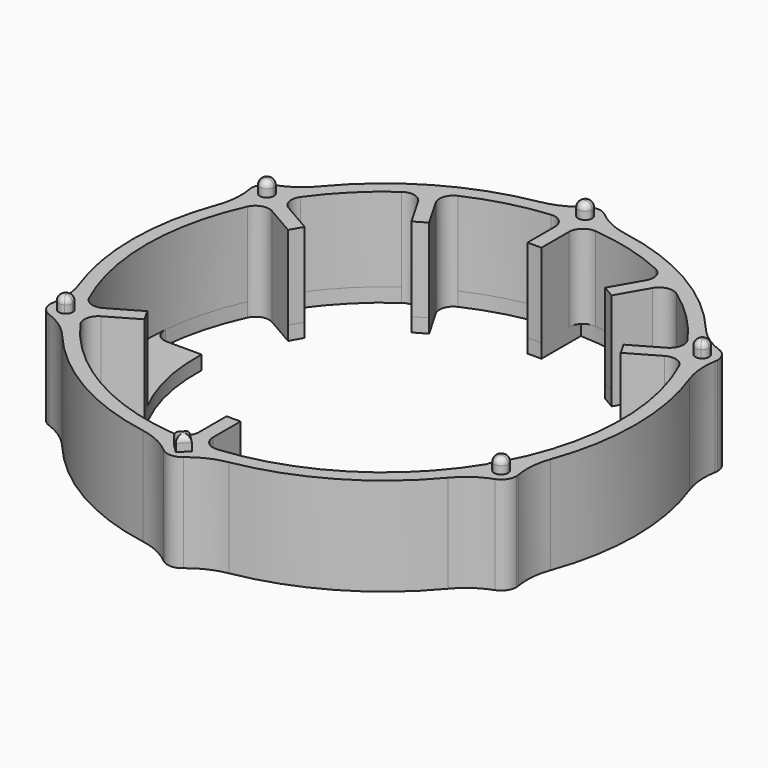
from build123d import *

# Parameters (mm, degrees)
F1_R         = 18
F1_R_2       = 17
F2_DEPTH     = 7
F3_DEPTH     = 7
F4_DEPTH     = 1
F6_DEPTH     = 7
F7_R         = 1
F8_R         = 5
F9_DEPTH     = 8
F10_R        = 0.44999
F11_DEPTH    = 1.8
F12_R        = 13.47
F13_DEPTH    = 1
F14_DEPTH    = 1
F15_T1_DEPTH = 3.7395798703
F15_T3_DEPTH = 1


# Not quite as in the source:
# - a fillet or chamfer that OpenCascade refuses, or shapes differently, is made with other operations: its cross-section is extruded or revolved along the edge and cut away or added
# - a fillet or chamfer is up to 0.001 mm smaller than in the source, because OpenCascade refuses the exact size
# - after a boolean that leaves OpenCascade's solid faulty, fix() repairs it


with BuildPart() as f2:
    # F1 (on Top) → F2 (new body)
    with BuildSketch(Plane.XY):
        Circle(F1_R)
        Circle(F1_R_2, mode=Mode.SUBTRACT)
    extrude(amount=F2_DEPTH)

    # F0 (on Top) → F3 (join)
    with BuildSketch(Plane.XY):
        with BuildLine():
            Line((-11.4073228059, 7.1633711619), (-14.4660626528, 8.9293354359))
            ThreePointArc((-14.4660626528, 8.9293354359), (-14.7224318643, 8.5), (-14.9660626528, 8.0633100321))
            Line((-14.9660626528, 8.0633100321), (-11.9073228059, 6.2973457581))
            ThreePointArc((-11.9073228059, 6.2973457581), (-11.665362189, 6.735), (-11.4073228059, 7.1633711619))
        make_face()
        with BuildLine():
            Line((7.1633711619, 11.4073228059), (8.9293354359, 14.4660626528))
            ThreePointArc((8.9293354359, 14.4660626528), (8.5, 14.7224318643), (8.0633100321, 14.9660626528))
            Line((8.0633100321, 14.9660626528), (6.2973457581, 11.9073228059))
            ThreePointArc((6.2973457581, 11.9073228059), (6.735, 11.665362189), (7.1633711619, 11.4073228059))
        make_face()
        with BuildLine():
            ThreePointArc((-0.5, -16.992645468), (0, -17), (0.5, -16.992645468))
            Line((0.5, -16.992645468), (0.5, -13.46071692))
            ThreePointArc((0.5, -13.46071692), (0, -13.47), (-0.5, -13.46071692))
            Line((-0.5, -13.46071692), (-0.5, -16.992645468))
        make_face()
        with BuildLine():
            ThreePointArc((-14.9660626528, -8.0633100321), (-14.7224318643, -8.5), (-14.4660626528, -8.9293354359))
            Line((-14.4660626528, -8.9293354359), (-11.4073228059, -7.1633711619))
            ThreePointArc((-11.4073228059, -7.1633711619), (-11.665362189, -6.735), (-11.9073228059, -6.2973457581))
            Line((-11.9073228059, -6.2973457581), (-14.9660626528, -8.0633100321))
        make_face()
        with BuildLine():
            Line((-6.2973457581, 11.9073228059), (-8.0633100321, 14.9660626528))
            ThreePointArc((-8.0633100321, 14.9660626528), (-8.5, 14.7224318643), (-8.9293354359, 14.4660626528))
            Line((-8.9293354359, 14.4660626528), (-7.1633711619, 11.4073228059))
            ThreePointArc((-7.1633711619, 11.4073228059), (-6.735, 11.665362189), (-6.2973457581, 11.9073228059))
        make_face()
        with BuildLine():
            Line((0.5, 13.46071692), (0.5, 16.992645468))
            ThreePointArc((0.5, 16.992645468), (0, 17), (-0.5, 16.992645468))
            Line((-0.5, 16.992645468), (-0.5, 13.46071692))
            ThreePointArc((-0.5, 13.46071692), (0, 13.47), (0.5, 13.46071692))
        make_face()
        with BuildLine():
            Line((11.9073228059, 6.2973457581), (14.9660626528, 8.0633100321))
            ThreePointArc((14.9660626528, 8.0633100321), (14.7224318643, 8.5), (14.4660626528, 8.9293354359))
            Line((14.4660626528, 8.9293354359), (11.4073228059, 7.1633711619))
            ThreePointArc((11.4073228059, 7.1633711619), (11.665362189, 6.735), (11.9073228059, 6.2973457581))
        make_face()
    extrude(amount=F3_DEPTH)

    # F1 (on Top) → F4 (join)
    with BuildSketch(Plane.XY):
        Circle(F1_R)
        Circle(F1_R_2, mode=Mode.SUBTRACT)
        Circle(F1_R_2)
    extrude(amount=F4_DEPTH)

    # F5 (on Top) → F6 (join)
    with BuildSketch(Plane.XY):
        with BuildLine():
            ThreePointArc((-14.4884572681, 9), (-14.6275367743, 9.5353800561), (-15.0096060035, 9.935377578))
            ThreePointArc((-15.0096060035, 9.935377578), (-15.1731450826, 9.6837837802), (-15.3324673166, 9.4294987133))
            ThreePointArc((-15.3324673166, 9.4294987133), (-15.153718855, 9.2469868663), (-15.0884572681, 9))
            ThreePointArc((-15.0884572681, 9), (-15.3354561915, 8.5687338928), (-15.832419089, 8.5635568422))
            ThreePointArc((-15.832419089, 8.5635568422), (-15.9729752997, 8.2984372068), (-16.1090923805, 8.0310113108))
            ThreePointArc((-16.1090923805, 8.0310113108), (-15.0239657375, 8.0558870238), (-14.4884572681, 9))
        make_face()
        with BuildLine():
            ThreePointArc((-15.3324673166, 9.4294987133), (-15.1731450826, 9.6837837802), (-15.0096060035, 9.935377578))
            ThreePointArc((-15.0096060035, 9.935377578), (-16.5410852123, 9.55), (-16.1090923805, 8.0310113108))
            ThreePointArc((-16.1090923805, 8.0310113108), (-15.9729752997, 8.2984372068), (-15.832419089, 8.5635568422))
            ThreePointArc((-15.832419089, 8.5635568422), (-16.02146997, 9.25), (-15.3324673166, 9.4294987133))
        make_face()
        with BuildLine():
            ThreePointArc((-1.099486377, 17.9663888889), (0, 16.9), (1.099486377, 17.9663888889))
            ThreePointArc((1.099486377, 17.9663888889), (0.7998302171, 17.982220987), (0.4999517724, 17.9930555556))
            ThreePointArc((0.4999517724, 17.9930555556), (0, 17.5), (-0.4999517724, 17.9930555556))
            ThreePointArc((-0.4999517724, 17.9930555556), (-0.7998302171, 17.982220987), (-1.099486377, 17.9663888889))
        make_face()
        with BuildLine():
            ThreePointArc((0.4999517724, 17.9930555556), (0.7998302171, 17.982220987), (1.099486377, 17.9663888889))
            ThreePointArc((1.099486377, 17.9663888889), (1.0998715868, 17.9831924823), (1.1, 18))
            ThreePointArc((1.1, 18), (-0.0168075177, 19.0998715868), (-1.099486377, 17.9663888889))
            ThreePointArc((-1.099486377, 17.9663888889), (-0.7998302171, 17.982220987), (-0.4999517724, 17.9930555556))
            ThreePointArc((-0.4999517724, 17.9930555556), (-0.003472306, 18.4999879429), (0.5, 18))
            ThreePointArc((0.5, 18), (0.4999879429, 17.996527694), (0.4999517724, 17.9930555556))
        make_face()
        with BuildLine():
            ThreePointArc((15.832419089, 8.5635568422), (15.9729752997, 8.2984372068), (16.1090923805, 8.0310113108))
            ThreePointArc((16.1090923805, 8.0310113108), (16.5325702443, 8.4355084694), (16.6884572681, 9))
            ThreePointArc((16.6884572681, 9), (16.1238373242, 9.9609204939), (15.0096060035, 9.935377578))
            ThreePointArc((15.0096060035, 9.935377578), (15.1731450826, 9.6837837802), (15.3324673166, 9.4294987133))
            ThreePointArc((15.3324673166, 9.4294987133), (15.8354441344, 9.4347384132), (16.0884572681, 9))
            ThreePointArc((16.0884572681, 9), (16.0197233753, 8.7469989234), (15.832419089, 8.5635568422))
        make_face()
        with BuildLine():
            ThreePointArc((15.0096060035, 9.935377578), (14.635829324, 8.45), (16.1090923805, 8.0310113108))
            ThreePointArc((16.1090923805, 8.0310113108), (15.9729752997, 8.2984372068), (15.832419089, 8.5635568422))
            ThreePointArc((15.832419089, 8.5635568422), (15.1554445662, 8.75), (15.3324673166, 9.4294987133))
            ThreePointArc((15.3324673166, 9.4294987133), (15.1731450826, 9.6837837802), (15.0096060035, 9.935377578))
        make_face()
        with BuildLine():
            ThreePointArc((-15.3324673166, -9.4294987133), (-15.1731450826, -9.6837837802), (-15.0096060035, -9.935377578))
            ThreePointArc((-15.0096060035, -9.935377578), (-14.6275367743, -9.5353800561), (-14.4884572681, -9))
            ThreePointArc((-14.4884572681, -9), (-15.0239657375, -8.0558870238), (-16.1090923805, -8.0310113108))
            ThreePointArc((-16.1090923805, -8.0310113108), (-15.9729752997, -8.2984372068), (-15.832419089, -8.5635568422))
            ThreePointArc((-15.832419089, -8.5635568422), (-15.3354561915, -8.5687338928), (-15.0884572681, -9))
            ThreePointArc((-15.0884572681, -9), (-15.153718855, -9.2469868663), (-15.3324673166, -9.4294987133))
        make_face()
        with BuildLine():
            ThreePointArc((-16.1090923805, -8.0310113108), (-16.5410852123, -9.55), (-15.0096060035, -9.935377578))
            ThreePointArc((-15.0096060035, -9.935377578), (-15.1731450826, -9.6837837802), (-15.3324673166, -9.4294987133))
            ThreePointArc((-15.3324673166, -9.4294987133), (-16.02146997, -9.25), (-15.832419089, -8.5635568422))
            ThreePointArc((-15.832419089, -8.5635568422), (-15.9729752997, -8.2984372068), (-16.1090923805, -8.0310113108))
        make_face()
        with BuildLine():
            ThreePointArc((0.6255239257, -17.9891278226), (0.8625800837, -17.9793202207), (1.099486377, -17.9663888889))
            ThreePointArc((1.099486377, -17.9663888889), (0, -16.9), (-1.099486377, -17.9663888889))
            ThreePointArc((-1.099486377, -17.9663888889), (-0.8625800837, -17.9793202207), (-0.6255239257, -17.9891278226))
            Line((-0.6255239257, -17.9891278226), (0, -17.3636038969))
            Line((0, -17.3636038969), (0.6255239257, -17.9891278226))
        make_face()
        with BuildLine():
            ThreePointArc((1.1, -18), (1.0998715868, -17.9831924823), (1.099486377, -17.9663888889))
            ThreePointArc((1.099486377, -17.9663888889), (0.8625800837, -17.9793202207), (0.6255239257, -17.9891278226))
            Line((0.6255239257, -17.9891278226), (0.6363961031, -18))
            Line((0.6363961031, -18), (0, -18.6363961031))
            Line((0, -18.6363961031), (-0.6363961031, -18))
            Line((-0.6363961031, -18), (-0.6255239257, -17.9891278226))
            ThreePointArc((-0.6255239257, -17.9891278226), (-0.8625800837, -17.9793202207), (-1.099486377, -17.9663888889))
            ThreePointArc((-1.099486377, -17.9663888889), (-0.0168075177, -19.0998715868), (1.1, -18))
        make_face()
        with BuildLine():
            ThreePointArc((16.6884572681, -9), (16.5325702443, -8.4355084694), (16.1090923805, -8.0310113108))
            ThreePointArc((16.1090923805, -8.0310113108), (15.9729752997, -8.2984372068), (15.832419089, -8.5635568422))
            ThreePointArc((15.832419089, -8.5635568422), (16.0197233753, -8.7469989234), (16.0884572681, -9))
            ThreePointArc((16.0884572681, -9), (15.8354441344, -9.4347384132), (15.3324673166, -9.4294987133))
            ThreePointArc((15.3324673166, -9.4294987133), (15.1731450826, -9.6837837802), (15.0096060035, -9.935377578))
            ThreePointArc((15.0096060035, -9.935377578), (16.1238373242, -9.9609204939), (16.6884572681, -9))
        make_face()
        with BuildLine():
            ThreePointArc((15.832419089, -8.5635568422), (15.9729752997, -8.2984372068), (16.1090923805, -8.0310113108))
            ThreePointArc((16.1090923805, -8.0310113108), (14.635829324, -8.45), (15.0096060035, -9.935377578))
            ThreePointArc((15.0096060035, -9.935377578), (15.1731450826, -9.6837837802), (15.3324673166, -9.4294987133))
            ThreePointArc((15.3324673166, -9.4294987133), (15.1554445662, -8.75), (15.832419089, -8.5635568422))
        make_face()
        with BuildLine():
            ThreePointArc((-15.0884572681, 9), (-15.153718855, 9.2469868663), (-15.3324673166, 9.4294987133))
            ThreePointArc((-15.3324673166, 9.4294987133), (-15.5884572681, 9), (-15.832419089, 8.5635568422))
            ThreePointArc((-15.832419089, 8.5635568422), (-15.3354561915, 8.5687338928), (-15.0884572681, 9))
        make_face()
        with BuildLine():
            ThreePointArc((-15.832419089, 8.5635568422), (-15.5884572681, 9), (-15.3324673166, 9.4294987133))
            ThreePointArc((-15.3324673166, 9.4294987133), (-16.02146997, 9.25), (-15.832419089, 8.5635568422))
        make_face()
        with BuildLine():
            ThreePointArc((-0.4999517724, 17.9930555556), (0, 18), (0.4999517724, 17.9930555556))
            ThreePointArc((0.4999517724, 17.9930555556), (0.4999879429, 17.996527694), (0.5, 18))
            ThreePointArc((0.5, 18), (-0.003472306, 18.4999879429), (-0.4999517724, 17.9930555556))
        make_face()
        with BuildLine():
            ThreePointArc((-0.4999517724, 17.9930555556), (0, 17.5), (0.4999517724, 17.9930555556))
            ThreePointArc((0.4999517724, 17.9930555556), (0, 18), (-0.4999517724, 17.9930555556))
        make_face()
        with BuildLine():
            ThreePointArc((15.3324673166, 9.4294987133), (15.5884572681, 9), (15.832419089, 8.5635568422))
            ThreePointArc((15.832419089, 8.5635568422), (16.0197233753, 8.7469989234), (16.0884572681, 9))
            ThreePointArc((16.0884572681, 9), (15.8354441344, 9.4347384132), (15.3324673166, 9.4294987133))
        make_face()
        with BuildLine():
            ThreePointArc((15.3324673166, 9.4294987133), (15.1554445662, 8.75), (15.832419089, 8.5635568422))
            ThreePointArc((15.832419089, 8.5635568422), (15.5884572681, 9), (15.3324673166, 9.4294987133))
        make_face()
        with BuildLine():
            ThreePointArc((16.0884572681, -9), (16.0197233753, -8.7469989234), (15.832419089, -8.5635568422))
            ThreePointArc((15.832419089, -8.5635568422), (15.5884572681, -9), (15.3324673166, -9.4294987133))
            ThreePointArc((15.3324673166, -9.4294987133), (15.8354441344, -9.4347384132), (16.0884572681, -9))
        make_face()
        with BuildLine():
            ThreePointArc((15.3324673166, -9.4294987133), (15.5884572681, -9), (15.832419089, -8.5635568422))
            ThreePointArc((15.832419089, -8.5635568422), (15.1554445662, -8.75), (15.3324673166, -9.4294987133))
        make_face()
        with BuildLine():
            Line((0.6363961031, -18), (0.6255239257, -17.9891278226))
            ThreePointArc((0.6255239257, -17.9891278226), (0, -18), (-0.6255239257, -17.9891278226))
            Line((-0.6255239257, -17.9891278226), (-0.6363961031, -18))
            Line((-0.6363961031, -18), (0, -18.6363961031))
            Line((0, -18.6363961031), (0.6363961031, -18))
        make_face()
        with BuildLine():
            ThreePointArc((-15.832419089, -8.5635568422), (-16.02146997, -9.25), (-15.3324673166, -9.4294987133))
            ThreePointArc((-15.3324673166, -9.4294987133), (-15.5884572681, -9), (-15.832419089, -8.5635568422))
        make_face()
        with BuildLine():
            ThreePointArc((-15.832419089, -8.5635568422), (-15.5884572681, -9), (-15.3324673166, -9.4294987133))
            ThreePointArc((-15.3324673166, -9.4294987133), (-15.153718855, -9.2469868663), (-15.0884572681, -9))
            ThreePointArc((-15.0884572681, -9), (-15.3354561915, -8.5687338928), (-15.832419089, -8.5635568422))
        make_face()
        with BuildLine():
            ThreePointArc((-0.6255239257, -17.9891278226), (0, -18), (0.6255239257, -17.9891278226))
            Line((0.6255239257, -17.9891278226), (0, -17.3636038969))
            Line((0, -17.3636038969), (-0.6255239257, -17.9891278226))
        make_face()
    extrude(amount=F6_DEPTH)

    # F7
    f7_edges = [f2.edges().sort_by_distance(p)[0] for p in [
        (0.5, -16.992645, 4),
        (8.06331, 14.966063, 4),
        (-14.966063, -8.06331, 4),
        (-8.06331, 14.966063, 4),
        (-14.466063, 8.929335, 4),
        (-0.5, 16.992645, 4),
        (14.466063, 8.929335, 4),
        (-14.966063, 8.06331, 4),
        (-8.929335, 14.466063, 4),
        (0.5, 16.992645, 4),
        (-14.466063, -8.929335, 4),
        (8.929335, 14.466063, 4),
        (14.966063, 8.06331, 4),
        (-0.5, -16.992645, 4),
    ]]
    fillet(f7_edges, radius=F7_R)

    # F8 (call 1 of 12: OpenCascade refuses the feature's edges together)
    f8_edges = [f2.edges().sort_by_distance(p)[0] for p in [
        (-16.109092, 8.031011, 3.5),
    ]]
    fillet(f8_edges, radius=F8_R)

    # F8#2 (call 2 of 12)
    f8_2_edges = [f2.edges().sort_by_distance(p)[0] for p in [
        (-15.009606, 9.935378, 3.5),
    ]]
    fillet(f8_2_edges, radius=F8_R)

    # F8#3 (call 3 of 12)
    f8_3_edges = [f2.edges().sort_by_distance(p)[0] for p in [
        (-1.099486, 17.966389, 3.5),
    ]]
    fillet(f8_3_edges, radius=F8_R)

    # F8#4 (call 4 of 12)
    f8_4_edges = [f2.edges().sort_by_distance(p)[0] for p in [
        (1.099486, 17.966389, 3.5),
    ]]
    fillet(f8_4_edges, radius=F8_R)

    # F8#5 (call 5 of 12)
    f8_5_edges = [f2.edges().sort_by_distance(p)[0] for p in [
        (-15.009606, -9.935378, 3.5),
    ]]
    fillet(f8_5_edges, radius=F8_R)

    # F8#6 (call 6 of 12)
    f8_6_edges = [f2.edges().sort_by_distance(p)[0] for p in [
        (-16.109092, -8.031011, 3.5),
    ]]
    fillet(f8_6_edges, radius=F8_R)

    # F8#7 (call 7 of 12)
    f8_7_edges = [f2.edges().sort_by_distance(p)[0] for p in [
        (1.099486, -17.966389, 3.5),
    ]]
    fillet(f8_7_edges, radius=F8_R)

    # F8#8 (call 8 of 12)
    f8_8_edges = [f2.edges().sort_by_distance(p)[0] for p in [
        (-1.099486, -17.966389, 3.5),
    ]]
    fillet(f8_8_edges, radius=F8_R)

    # F8#10 (call 9 of 12)
    f8_10_edges = [f2.edges().sort_by_distance(p)[0] for p in [
        (15.009606, -9.935378, 3.5),
    ]]
    fillet(f8_10_edges, radius=F8_R)

    # F8#11 (call 10 of 12)
    f8_11_edges = [f2.edges().sort_by_distance(p)[0] for p in [
        (16.109092, 8.031011, 3.5),
    ]]
    fillet(f8_11_edges, radius=F8_R)

    # F8#12 (call 11 of 12)
    f8_12_edges = [f2.edges().sort_by_distance(p)[0] for p in [
        (15.009606, 9.935378, 3.5),
    ]]
    fillet(f8_12_edges, radius=F8_R)

    # F8#9 (call 12 of 12)
    f8_9_edges = [f2.edges().sort_by_distance(p)[0] for p in [
        (16.109092, -8.031011, 3.5),
    ]]
    fillet(f8_9_edges, radius=F8_R)

    # F5 (on Top) → F9 (join)
    with BuildSketch(Plane.XY):
        with BuildLine():
            ThreePointArc((-15.832419089, 8.5635568422), (-15.5884572681, 9), (-15.3324673166, 9.4294987133))
            ThreePointArc((-15.3324673166, 9.4294987133), (-16.02146997, 9.25), (-15.832419089, 8.5635568422))
        make_face()
        with BuildLine():
            ThreePointArc((-15.0884572681, 9), (-15.153718855, 9.2469868663), (-15.3324673166, 9.4294987133))
            ThreePointArc((-15.3324673166, 9.4294987133), (-15.5884572681, 9), (-15.832419089, 8.5635568422))
            ThreePointArc((-15.832419089, 8.5635568422), (-15.3354561915, 8.5687338928), (-15.0884572681, 9))
        make_face()
        with BuildLine():
            ThreePointArc((-0.4999517724, 17.9930555556), (0, 18), (0.4999517724, 17.9930555556))
            ThreePointArc((0.4999517724, 17.9930555556), (0.4999879429, 17.996527694), (0.5, 18))
            ThreePointArc((0.5, 18), (-0.003472306, 18.4999879429), (-0.4999517724, 17.9930555556))
        make_face()
        with BuildLine():
            ThreePointArc((-0.4999517724, 17.9930555556), (0, 17.5), (0.4999517724, 17.9930555556))
            ThreePointArc((0.4999517724, 17.9930555556), (0, 18), (-0.4999517724, 17.9930555556))
        make_face()
        with BuildLine():
            ThreePointArc((15.3324673166, 9.4294987133), (15.1554445662, 8.75), (15.832419089, 8.5635568422))
            ThreePointArc((15.832419089, 8.5635568422), (15.5884572681, 9), (15.3324673166, 9.4294987133))
        make_face()
        with BuildLine():
            ThreePointArc((15.3324673166, 9.4294987133), (15.5884572681, 9), (15.832419089, 8.5635568422))
            ThreePointArc((15.832419089, 8.5635568422), (16.0197233753, 8.7469989234), (16.0884572681, 9))
            ThreePointArc((16.0884572681, 9), (15.8354441344, 9.4347384132), (15.3324673166, 9.4294987133))
        make_face()
        with BuildLine():
            ThreePointArc((15.3324673166, -9.4294987133), (15.5884572681, -9), (15.832419089, -8.5635568422))
            ThreePointArc((15.832419089, -8.5635568422), (15.1554445662, -8.75), (15.3324673166, -9.4294987133))
        make_face()
        with BuildLine():
            ThreePointArc((16.0884572681, -9), (16.0197233753, -8.7469989234), (15.832419089, -8.5635568422))
            ThreePointArc((15.832419089, -8.5635568422), (15.5884572681, -9), (15.3324673166, -9.4294987133))
            ThreePointArc((15.3324673166, -9.4294987133), (15.8354441344, -9.4347384132), (16.0884572681, -9))
        make_face()
        with BuildLine():
            Line((0.6363961031, -18), (0.6255239257, -17.9891278226))
            ThreePointArc((0.6255239257, -17.9891278226), (0, -18), (-0.6255239257, -17.9891278226))
            Line((-0.6255239257, -17.9891278226), (-0.6363961031, -18))
            Line((-0.6363961031, -18), (0, -18.6363961031))
            Line((0, -18.6363961031), (0.6363961031, -18))
        make_face()
        with BuildLine():
            ThreePointArc((-0.6255239257, -17.9891278226), (0, -18), (0.6255239257, -17.9891278226))
            Line((0.6255239257, -17.9891278226), (0, -17.3636038969))
            Line((0, -17.3636038969), (-0.6255239257, -17.9891278226))
        make_face()
        with BuildLine():
            ThreePointArc((-15.832419089, -8.5635568422), (-16.02146997, -9.25), (-15.3324673166, -9.4294987133))
            ThreePointArc((-15.3324673166, -9.4294987133), (-15.5884572681, -9), (-15.832419089, -8.5635568422))
        make_face()
        with BuildLine():
            ThreePointArc((-15.832419089, -8.5635568422), (-15.5884572681, -9), (-15.3324673166, -9.4294987133))
            ThreePointArc((-15.3324673166, -9.4294987133), (-15.153718855, -9.2469868663), (-15.0884572681, -9))
            ThreePointArc((-15.0884572681, -9), (-15.3354561915, -8.5687338928), (-15.832419089, -8.5635568422))
        make_face()
    extrude(amount=F9_DEPTH)

    # F10 (radius 0.45 in the source; OpenCascade refuses exactly that, so slightly less here)
    f10_edges = [f2.edges().sort_by_distance(p)[0] for p in [
        (-15.844447, -8.570501, 8),
        (-15.344495, 9.436443, 8),
        (0.499952, 18.006944, 8),
        (15.344495, 9.436443, 8),
        (15.844447, -8.570501, 8),
        (0.318198, -17.681802, 8),
        (-0.318198, -18.318198, 8),
        (0.318198, -18.318198, 8),
        (-0.318198, -17.681802, 8),
    ]]
    fillet(f10_edges, radius=F10_R)

    # F5 (on Top) → F11 (cut)
    with BuildSketch(Plane.XY):
        with BuildLine():
            ThreePointArc((-15.832419089, -8.5635568422), (-16.02146997, -9.25), (-15.3324673166, -9.4294987133))
            ThreePointArc((-15.3324673166, -9.4294987133), (-15.5884572681, -9), (-15.832419089, -8.5635568422))
        make_face()
        with BuildLine():
            ThreePointArc((-15.832419089, -8.5635568422), (-15.5884572681, -9), (-15.3324673166, -9.4294987133))
            ThreePointArc((-15.3324673166, -9.4294987133), (-15.153718855, -9.2469868663), (-15.0884572681, -9))
            ThreePointArc((-15.0884572681, -9), (-15.3354561915, -8.5687338928), (-15.832419089, -8.5635568422))
        make_face()
        with BuildLine():
            Line((0.6363961031, -18), (0.6255239257, -17.9891278226))
            ThreePointArc((0.6255239257, -17.9891278226), (0, -18), (-0.6255239257, -17.9891278226))
            Line((-0.6255239257, -17.9891278226), (-0.6363961031, -18))
            Line((-0.6363961031, -18), (0, -18.6363961031))
            Line((0, -18.6363961031), (0.6363961031, -18))
        make_face()
        with BuildLine():
            ThreePointArc((-0.6255239257, -17.9891278226), (0, -18), (0.6255239257, -17.9891278226))
            Line((0.6255239257, -17.9891278226), (0, -17.3636038969))
            Line((0, -17.3636038969), (-0.6255239257, -17.9891278226))
        make_face()
        with BuildLine():
            ThreePointArc((15.3324673166, -9.4294987133), (15.5884572681, -9), (15.832419089, -8.5635568422))
            ThreePointArc((15.832419089, -8.5635568422), (15.1554445662, -8.75), (15.3324673166, -9.4294987133))
        make_face()
        with BuildLine():
            ThreePointArc((16.0884572681, -9), (16.0197233753, -8.7469989234), (15.832419089, -8.5635568422))
            ThreePointArc((15.832419089, -8.5635568422), (15.5884572681, -9), (15.3324673166, -9.4294987133))
            ThreePointArc((15.3324673166, -9.4294987133), (15.8354441344, -9.4347384132), (16.0884572681, -9))
        make_face()
        with BuildLine():
            ThreePointArc((15.3324673166, 9.4294987133), (15.1554445662, 8.75), (15.832419089, 8.5635568422))
            ThreePointArc((15.832419089, 8.5635568422), (15.5884572681, 9), (15.3324673166, 9.4294987133))
        make_face()
        with BuildLine():
            ThreePointArc((15.3324673166, 9.4294987133), (15.5884572681, 9), (15.832419089, 8.5635568422))
            ThreePointArc((15.832419089, 8.5635568422), (16.0197233753, 8.7469989234), (16.0884572681, 9))
            ThreePointArc((16.0884572681, 9), (15.8354441344, 9.4347384132), (15.3324673166, 9.4294987133))
        make_face()
        with BuildLine():
            ThreePointArc((-0.4999517724, 17.9930555556), (0, 17.5), (0.4999517724, 17.9930555556))
            ThreePointArc((0.4999517724, 17.9930555556), (0, 18), (-0.4999517724, 17.9930555556))
        make_face()
        with BuildLine():
            ThreePointArc((-0.4999517724, 17.9930555556), (0, 18), (0.4999517724, 17.9930555556))
            ThreePointArc((0.4999517724, 17.9930555556), (0.4999879429, 17.996527694), (0.5, 18))
            ThreePointArc((0.5, 18), (-0.003472306, 18.4999879429), (-0.4999517724, 17.9930555556))
        make_face()
        with BuildLine():
            ThreePointArc((-15.832419089, 8.5635568422), (-15.5884572681, 9), (-15.3324673166, 9.4294987133))
            ThreePointArc((-15.3324673166, 9.4294987133), (-16.02146997, 9.25), (-15.832419089, 8.5635568422))
        make_face()
        with BuildLine():
            ThreePointArc((-15.0884572681, 9), (-15.153718855, 9.2469868663), (-15.3324673166, 9.4294987133))
            ThreePointArc((-15.3324673166, 9.4294987133), (-15.5884572681, 9), (-15.832419089, 8.5635568422))
            ThreePointArc((-15.832419089, 8.5635568422), (-15.3354561915, 8.5687338928), (-15.0884572681, 9))
        make_face()
    extrude(amount=F11_DEPTH, mode=Mode.SUBTRACT)

    # F12 (on Top) → F13 (cut)
    with BuildSketch(Plane.XY):
        Circle(F12_R)
    extrude(amount=F13_DEPTH, mode=Mode.SUBTRACT)

    add(f2.part.fix(), mode=Mode.REPLACE)

    # F0 (on Top) → F14 (cut)
    with BuildSketch(Plane.XY):
        with BuildLine():
            ThreePointArc((8.9293354359, -14.4660626528), (12.0208152802, -12.0208152802), (14.4660626528, -8.9293354359))
            Line((14.4660626528, -8.9293354359), (11.4073228059, -7.1633711619))
            ThreePointArc((11.4073228059, -7.1633711619), (9.5247283426, -9.5247283426), (7.1633711619, -11.4073228059))
            Line((7.1633711619, -11.4073228059), (8.9293354359, -14.4660626528))
        make_face()
        with BuildLine():
            Line((11.4073228059, 7.1633711619), (14.4660626528, 8.9293354359))
            ThreePointArc((14.4660626528, 8.9293354359), (12.0208152802, 12.0208152802), (8.9293354359, 14.4660626528))
            Line((8.9293354359, 14.4660626528), (7.1633711619, 11.4073228059))
            ThreePointArc((7.1633711619, 11.4073228059), (9.5247283426, 9.5247283426), (11.4073228059, 7.1633711619))
        make_face()
        with BuildLine():
            Line((6.2973457581, 11.9073228059), (8.0633100321, 14.9660626528))
            ThreePointArc((8.0633100321, 14.9660626528), (4.3999237667, 16.4207390469), (0.5, 16.992645468))
            Line((0.5, 16.992645468), (0.5, 13.46071692))
            ThreePointArc((0.5, 13.46071692), (3.4862925375, 13.0110208801), (6.2973457581, 11.9073228059))
        make_face()
        with BuildLine():
            Line((-0.5, 13.46071692), (-0.5, 16.992645468))
            ThreePointArc((-0.5, 16.992645468), (-4.3999237667, 16.4207390469), (-8.0633100321, 14.9660626528))
            Line((-8.0633100321, 14.9660626528), (-6.2973457581, 11.9073228059))
            ThreePointArc((-6.2973457581, 11.9073228059), (-3.4862925375, 13.0110208801), (-0.5, 13.46071692))
        make_face()
        with BuildLine():
            Line((-7.1633711619, 11.4073228059), (-8.9293354359, 14.4660626528))
            ThreePointArc((-8.9293354359, 14.4660626528), (-12.0208152802, 12.0208152802), (-14.4660626528, 8.9293354359))
            Line((-14.4660626528, 8.9293354359), (-11.4073228059, 7.1633711619))
            ThreePointArc((-11.4073228059, 7.1633711619), (-9.5247283426, 9.5247283426), (-7.1633711619, 11.4073228059))
        make_face()
        with BuildLine():
            Line((-11.9073228059, 6.2973457581), (-14.9660626528, 8.0633100321))
            ThreePointArc((-14.9660626528, 8.0633100321), (-16.4207390469, 4.3999237667), (-16.992645468, 0.5))
            Line((-16.992645468, 0.5), (-13.46071692, 0.5))
            ThreePointArc((-13.46071692, 0.5), (-13.0110208801, 3.4862925375), (-11.9073228059, 6.2973457581))
        make_face()
        with BuildLine():
            ThreePointArc((-14.4660626528, -8.9293354359), (-12.0208152802, -12.0208152802), (-8.9293354359, -14.4660626528))
            Line((-8.9293354359, -14.4660626528), (-7.1633711619, -11.4073228059))
            ThreePointArc((-7.1633711619, -11.4073228059), (-9.5247283426, -9.5247283426), (-11.4073228059, -7.1633711619))
            Line((-11.4073228059, -7.1633711619), (-14.4660626528, -8.9293354359))
        make_face()
    extrude(amount=F14_DEPTH, mode=Mode.SUBTRACT)

    # F15: fillet of radius 1 on 13 edges, made by hand

    # F15_s2 → F15_t1 (join)
    with BuildSketch(Plane.XY):
        with BuildLine():
            ThreePointArc((-15.4544658902, 7.0823360588), (-14.8492412837, 7.6184442326), (-14.0453796613, 7.5317534591))
            Line((-14.0453796613, 7.5317534591), (-14.9660626528, 8.0633100321))
            ThreePointArc((-14.9660626528, 8.0633100321), (-15.2181706092, 7.57675942), (-15.4544658902, 7.0823360588))
        make_face()
        with BuildLine():
            ThreePointArc((-9.8427920334, 13.8607158902), (-9.0505980623, 14.0223868846), (-8.3977788629, 13.5453796613))
            Line((-8.3977788629, 13.5453796613), (-8.9293354359, 14.4660626528))
            ThreePointArc((-8.9293354359, 14.4660626528), (-9.3909426367, 14.1707514407), (-9.8427920334, 13.8607158902))
        make_face()
        with BuildLine():
            ThreePointArc((8.3977788629, 13.5453796613), (9.0505980623, 14.0223868846), (9.8427920334, 13.8607158902))
            ThreePointArc((9.8427920334, 13.8607158902), (9.3909426367, 14.1707514407), (8.9293354359, 14.4660626528))
            Line((8.9293354359, 14.4660626528), (8.3977788629, 13.5453796613))
        make_face()
        with BuildLine():
            ThreePointArc((-13.5453796613, 8.3977788629), (-14.0223868846, 9.0505980623), (-13.8607158902, 9.8427920334))
            ThreePointArc((-13.8607158902, 9.8427920334), (-14.1707514407, 9.3909426367), (-14.4660626528, 8.9293354359))
            Line((-14.4660626528, 8.9293354359), (-13.5453796613, 8.3977788629))
        make_face()
        with BuildLine():
            ThreePointArc((-7.5317534591, 14.0453796613), (-7.6184442326, 14.8492412838), (-7.0823360588, 15.4544658902))
            ThreePointArc((-7.0823360588, 15.4544658902), (-7.57675942, 15.2181706092), (-8.0633100321, 14.9660626528))
            Line((-8.0633100321, 14.9660626528), (-7.5317534591, 14.0453796613))
        make_face()
        with BuildLine():
            ThreePointArc((-1.59375, 16.9251280922), (-0.8268543991, 16.669042295), (-0.5, 15.9295323221))
            Line((-0.5, 15.9295323221), (-0.5, 16.992645468))
            ThreePointArc((-0.5, 16.992645468), (-1.0474191685, 16.9677020567), (-1.59375, 16.9251280922))
        make_face()
        with BuildLine():
            ThreePointArc((7.0823360588, 15.4544658902), (7.6184442326, 14.8492412837), (7.5317534591, 14.0453796613))
            Line((7.5317534591, 14.0453796613), (8.0633100321, 14.9660626528))
            ThreePointArc((8.0633100321, 14.9660626528), (7.57675942, 15.2181706092), (7.0823360588, 15.4544658902))
        make_face()
        with BuildLine():
            ThreePointArc((13.8607158902, 9.8427920334), (14.0223868846, 9.0505980623), (13.5453796613, 8.3977788629))
            Line((13.5453796613, 8.3977788629), (14.4660626528, 8.9293354359))
            ThreePointArc((14.4660626528, 8.9293354359), (14.1707514407, 9.3909426367), (13.8607158902, 9.8427920334))
        make_face()
        with BuildLine():
            ThreePointArc((-13.8607158902, -9.8427920334), (-14.0223868846, -9.0505980623), (-13.5453796613, -8.3977788629))
            Line((-13.5453796613, -8.3977788629), (-14.4660626528, -8.9293354359))
            ThreePointArc((-14.4660626528, -8.9293354359), (-14.1707514407, -9.3909426367), (-13.8607158902, -9.8427920334))
        make_face()
    extrude(amount=F15_T1_DEPTH)

    # F15_s4 → F15_t3 (join)
    with BuildSketch(Plane.XY):
        with BuildLine():
            ThreePointArc((-16.9251280922, 1.59375), (-16.669042295, 0.8268543991), (-15.9295323221, 0.5))
            Line((-15.9295323221, 0.5), (-16.992645468, 0.5))
            ThreePointArc((-16.992645468, 0.5), (-16.9677020567, 1.0474191685), (-16.9251280922, 1.59375))
        make_face()
        with BuildLine():
            ThreePointArc((-9.8427920334, -13.8607158902), (-9.0505980623, -14.0223868846), (-8.3977788629, -13.5453796613))
            Line((-8.3977788629, -13.5453796613), (-8.9293354359, -14.4660626528))
            ThreePointArc((-8.9293354359, -14.4660626528), (-9.3909426367, -14.1707514407), (-9.8427920334, -13.8607158902))
        make_face()
        with BuildLine():
            ThreePointArc((9.8427920334, -13.8607158902), (9.0505980623, -14.0223868846), (8.3977788629, -13.5453796613))
            Line((8.3977788629, -13.5453796613), (8.9293354359, -14.4660626528))
            ThreePointArc((8.9293354359, -14.4660626528), (9.3909426367, -14.1707514407), (9.8427920334, -13.8607158902))
        make_face()
        with BuildLine():
            ThreePointArc((13.8607158902, -9.8427920334), (14.0223868846, -9.0505980623), (13.5453796613, -8.3977788629))
            Line((13.5453796613, -8.3977788629), (14.4660626528, -8.9293354359))
            ThreePointArc((14.4660626528, -8.9293354359), (14.1707514407, -9.3909426367), (13.8607158902, -9.8427920334))
        make_face()
    extrude(amount=F15_T3_DEPTH)


solid = f2.part
